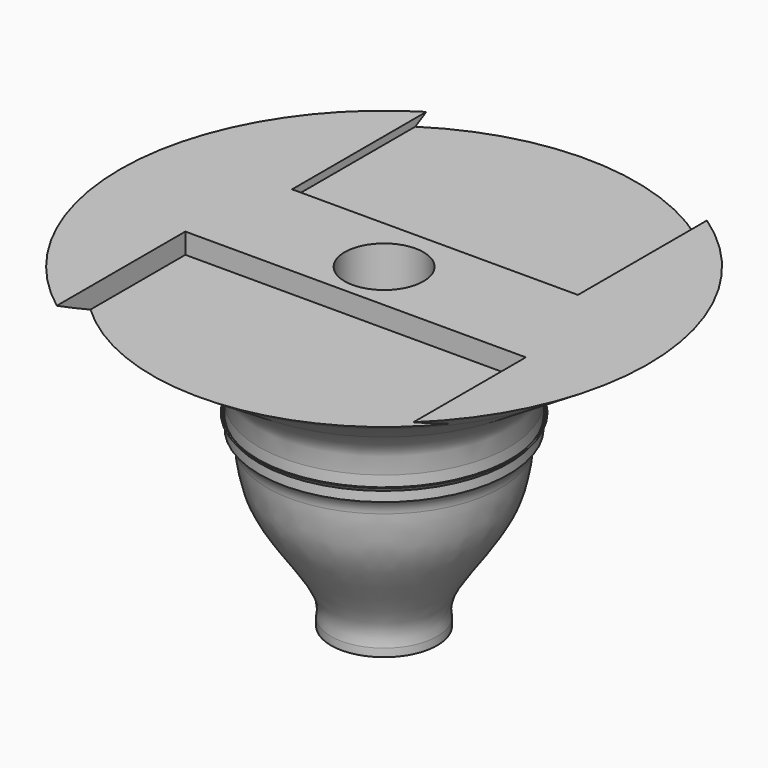
from build123d import *

# Parameters (mm, degrees)
F3_R     = 9.7677281956
F3_R_2   = 7.6796646
F4_DEPTH = 86.2554833293
F5_DEPTH = 1.8415
F6_DEPTH = 5.08


# Not quite as in the source:
# - a fillet or chamfer that OpenCascade refuses, or shapes differently, is made with other operations: its cross-section is extruded or revolved along the edge and cut away or added


with BuildPart() as f1:
    # F0 (on Front) → F1 (revolve)
    with BuildSketch(Plane.XZ):
        with BuildLine():
            add(Edge.make_bspline(
                [(-16.0994362086, 126.6403571513), (-15.4416487906, 129.818912005), (-18.3602187314, 137.0481581434), (-30.7776463133, 151.6944538615), (-31.8157197837, 162.4649808678), (-32.0365097363, 167.6998246302)],
                knots=[0, 0, 0, 0, 0.2764092674, 0.6542388522, 1, 1, 1, 1], degree=3))
            Line((-16.0994362086, 126.6403571513), (-16.0994362086, 124.6616938849))
            Line((-16.0994362086, 124.6616938849), (-10.6212262798, 124.6616938849))
            Line((-10.6212262798, 124.6616938849), (-10.6212262798, 126.6403571513))
            Line((-10.6212262798, 126.6403571513), (-10.6212262798, 167.9538246302))
            Line((-10.6212262798, 167.9538246302), (-10.6212262798, 173.5984517965))
            Line((-10.6212262798, 173.5984517965), (-10.6212262798, 192.7077323198))
            Line((-10.6212262798, 192.7077323198), (-10.6212262798, 202.9486296068))
            Line((-10.6212262798, 202.9486296068), (-68.306534248, 202.9486296068))
            Line((-68.306534248, 202.9486296068), (-56.8935275078, 195.6928223372))
            Line((-56.8935275078, 195.6928223372), (-41.0592220724, 185.6261789799))
            add(Edge.make_bspline(
                [(-33.8192135096, 173.5984517965), (-33.9311976843, 175.7700643461), (-34.1712077818, 180.4243736831), (-38.663140823, 183.8166663782), (-41.0592220724, 185.6261789799)],
                knots=[0, 0, 0, 0, 0.4665812951, 1, 1, 1, 1], degree=3))
            Line((-33.8192135096, 173.5984517965), (-33.8192135096, 170.823040801))
            Line((-33.8192135096, 170.823040801), (-33.8192135096, 170.6639382431))
            Line((-33.8192135096, 170.6639382431), (-34.1753996909, 171.1073964834))
            Line((-34.1753996909, 171.1073964834), (-34.47479508, 171.1073964834))
            Line((-34.47479508, 171.1073964834), (-34.5564074814, 171.1073964834))
            Line((-34.5564074814, 171.1073964834), (-33.8073261082, 170.1312959194))
            Line((-33.8073261082, 170.1312959194), (-33.8073261082, 167.6998246302))
            Line((-33.8073261082, 167.6998246302), (-32.0365097363, 167.6998246302))
        make_face()
    revolve(axis=Axis((-2.9415616798, 0, 150.6240181996), (0, 0, 1)))

    # F2: fillet of radius 5.08 on 1 edges, made by hand

    # F2_s1 → F2_t2 (revolve)
    with BuildSketch(Plane.XZ):
        with BuildLine():
            ThreePointArc((-31.8196671786, 164.0759580259), (-32.4282830228, 166.0991776077), (-33.8073261082, 167.6998246302))
            Line((-33.8073261082, 167.6998246302), (-33.7458267391, 167.780697293))
            ThreePointArc((-33.7458267391, 167.780697293), (-32.9219179223, 167.8014246302), (-32.0365097363, 167.8014246302))
            Line((-32.0365097363, 167.8014246302), (-31.934999984, 167.704106006))
            ThreePointArc((-31.934999984, 167.704106006), (-31.8450405903, 165.8927492145), (-31.7184146309, 164.0843533567))
            Line((-31.7184146309, 164.0843533567), (-31.8196671786, 164.0759580259))
        make_face()
    revolve(axis=Axis((-2.9415616798, 0, 167.6998246302), (0, 0, 1)))

    # F3 (on face) → F4 (cut)
    with BuildSketch(Plane.XY.offset(202.9486296068)):
        with Locations((-2.9415616798, 0)):
            Circle(F3_R)
        with Locations((-2.9415616798, 0)):
            Circle(F3_R_2, mode=Mode.SUBTRACT)
    extrude(amount=-F4_DEPTH, mode=Mode.SUBTRACT)

    # F3 (on face) → F5 (cut)
    with BuildSketch(Plane.XY.offset(202.9486296068)):
        with BuildLine():
            Line((-37.0871919824, 14.1988984612), (33.7026080176, 14.1988984612))
            Line((33.7026080176, 14.1988984612), (33.7026080176, 54.127483463))
            ThreePointArc((33.7026080176, 54.127483463), (-1.4554201029, 65.3480758864), (-37.0871919824, 55.7373803661))
            Line((-37.0871919824, 55.7373803661), (-37.0871919824, 14.1988984612))
        make_face()
    extrude(amount=-F5_DEPTH, mode=Mode.SUBTRACT)

    # F3 (on face) → F6 (cut)
    with BuildSketch(Plane.XY.offset(202.9486296068)):
        with BuildLine():
            Line((-42.164, -12.5023329654), (-42.164, -52.2893867918))
            ThreePointArc((-42.164, -52.2893867918), (0.9127584674, -65.2512364254), (42.164, -47.3082227989))
            Line((42.164, -47.3082227989), (42.164, -12.5023329654))
            Line((42.164, -12.5023329654), (-42.164, -12.5023329654))
        make_face()
    extrude(amount=-F6_DEPTH, mode=Mode.SUBTRACT)


solid = f1.part
